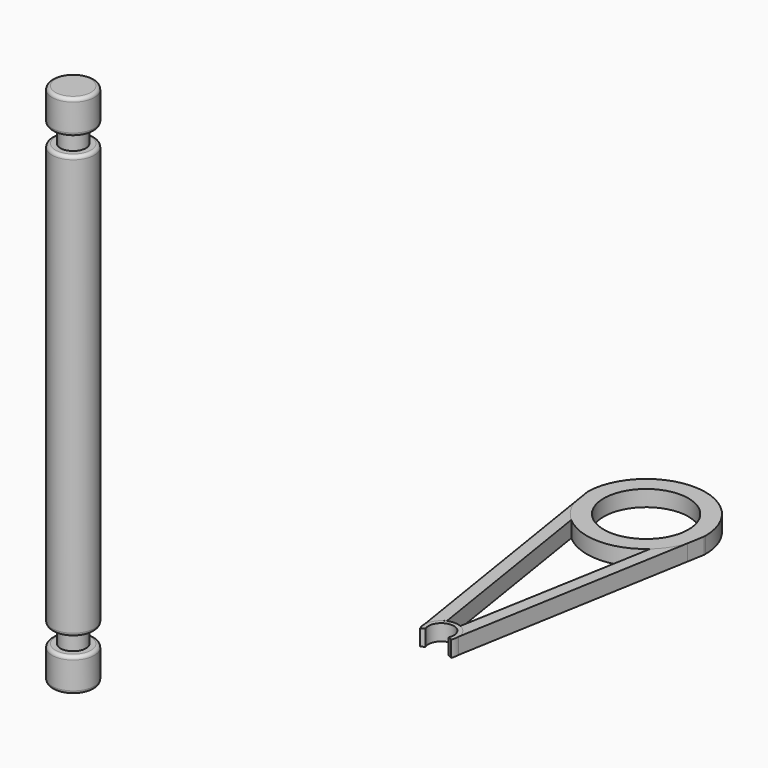
from build123d import *

# Parameters (mm, degrees)
F0_R      = 1.25
F1_DEPTH  = 25
F2_R      = 0.75
F3_DEPTH  = 1
F4_R      = 1.25
F5_DEPTH  = 2
F6_R      = 0.2
F7_R      = 0.75
F8_DEPTH  = 1
F9_R      = 1.25
F10_DEPTH = 2
F11_R     = 0.2
F14_DEPTH = 0.95
F13_R     = 2.5
F15_DEPTH = 0.95


# Not quite as in the source:
# - a feature names something its author has since deleted; it is built from what else it names


with BuildPart() as f1:
    # F0 (on Top) → F1 (new body)
    with BuildSketch(Plane.XY):
        with Locations((-14.0540208668, 1.2765177526)):
            Circle(F0_R)
    extrude(amount=F1_DEPTH)

    # F2 (on face) → F3 (join)
    with BuildSketch(Plane.XY.offset(25)):
        with Locations((-14.0540208668, 1.2765177526)):
            Circle(F2_R)
    extrude(amount=F3_DEPTH)

    # F4 (on face) → F5 (join)
    with BuildSketch(Plane.XY.offset(26)):
        with Locations((-14.0540208668, 1.2765177526)):
            Circle(F4_R)
    extrude(amount=F5_DEPTH)

    # F6
    f6_edges = [f1.edges().sort_by_distance(p)[0] for p in [
        (-15.304021, 1.276518, 25),
        (-15.304021, 1.276518, 26),
        (-15.304021, 1.276518, 28),
        (-15.304021, 1.276518, 0),
    ]]
    fillet(f6_edges, radius=F6_R)

    # F7 (on face) → F8 (join)
    with BuildSketch(Plane(origin=(0, 0, 0), x_dir=(1, 0, 0), z_dir=(0, 0, -1))):
        with Locations((-14.0540208668, -1.2765177526)):
            Circle(F7_R)
    extrude(amount=F8_DEPTH)

    # F9 (on face) → F10 (join)
    with BuildSketch(Plane(origin=(0, 0, -1), x_dir=(1, 0, 0), z_dir=(0, 0, -1))):
        with Locations((-14.0540208668, -1.2765177526)):
            Circle(F9_R)
    extrude(amount=F10_DEPTH)

    # F11
    f11_edges = [f1.edges().sort_by_distance(p)[0] for p in [
        (-15.304021, 1.276518, -3),
        (-15.304021, 1.276518, -1),
    ]]
    fillet(f11_edges, radius=F11_R)


with BuildPart() as f14:
    # F12 (on Top) → F14 (new body)
    with BuildSketch(Plane.XY):
        with BuildLine():
            ThreePointArc((0, 9.754398472), (0.718912718, 10.7180910171), (1.4378254361, 9.754398472))
            Line((1.4378254361, 9.754398472), (1.6326663215, 9.5595575866))
            ThreePointArc((1.6326663215, 9.5595575866), (0.7185053455, 10.9681246644), (-0.1951614716, 9.5592370004))
            Line((-0.1951614716, 9.5592370004), (0, 9.754398472))
        make_face()
    extrude(amount=F14_DEPTH)


with BuildPart() as f14b:
    # F13 (on face) → F14, piece 2 (new body)
    with BuildSketch(Plane.XY):
        with BuildLine():
            ThreePointArc((4.3177234546, 24.8866700044), (4.3184676742, 24.9283358265), (4.3187157592, 24.9700075561))
            ThreePointArc((4.3187157592, 24.9700075561), (0.8603874888, 28.4697594712), (-2.6802919362, 25.0533451079))
            Line((-2.6802919362, 25.0533451079), (-2.4813634191, 23.8040412543))
            ThreePointArc((-2.4813634191, 23.8040412543), (-2.0864758559, 23.0181208586), (-1.5081208042, 22.3554652239))
            ThreePointArc((-1.5081208042, 22.3554652239), (0.8187157592, 21.4700075561), (3.1455523226, 22.3554652239))
            ThreePointArc((3.1455523226, 22.3554652239), (3.7413801422, 23.044382228), (4.1392738139, 23.863710035))
            Line((4.1392738139, 23.863710035), (4.3177234546, 24.8866700044))
        make_face()
        with Locations((0.8187157592, 24.9700075561)):
            Circle(F13_R, mode=Mode.SUBTRACT)
    extrude(amount=F14_DEPTH)


with BuildPart() as f14c:
    # F13 (on face) → F14, piece 3 (new body)
    with BuildSketch(Plane.XY):
        Polygon((0, 9.754398472), (-0.1951614716, 9.5592370004), (0.0334535479, 9.6658419348), align=None)
    extrude(amount=F14_DEPTH)


with BuildPart() as f14d:
    # F13 (on face) → F14, piece 4 (new body)
    with BuildSketch(Plane.XY):
        Polygon((1.4058124998, 9.6653412609), (1.6326663215, 9.5595575866), (1.4378254361, 9.754398472), align=None)
    extrude(amount=F14_DEPTH)


with BuildPart() as f15:
    # F13 (on face) → F15 (new body)
    with BuildSketch(Plane.XY):
        with BuildLine():
            ThreePointArc((-1.5081208042, 22.3554652239), (-2.0864758559, 23.0181208586), (-2.4813634191, 23.8040412543))
            Line((-2.4813634191, 23.8040412543), (-0.281858813, 9.9907900398))
            ThreePointArc((-0.281858813, 9.9907900398), (-0.1121579443, 10.5252860826), (0.3184033106, 10.8845929296))
            Line((0.3184033106, 10.8845929296), (-1.5081208042, 22.3554652239))
        make_face()
    extrude(amount=F15_DEPTH)


with BuildPart() as f15b:
    # F13 (on face) → F15, piece 2 (new body)
    with BuildSketch(Plane.XY):
        with BuildLine():
            Line((1.7192205738, 9.9907900398), (4.1392738139, 23.863710035))
            ThreePointArc((4.1392738139, 23.863710035), (3.7413801422, 23.044382228), (3.1455523226, 22.3554652239))
            Line((3.1455523226, 22.3554652239), (1.1189584502, 10.8845929296))
            ThreePointArc((1.1189584502, 10.8845929296), (1.5495197052, 10.5252860826), (1.7192205738, 9.9907900398))
        make_face()
    extrude(amount=F15_DEPTH)


solid = Compound([f1.part, f14.part, f14b.part, f14c.part, f14d.part, f15.part, f15b.part])
